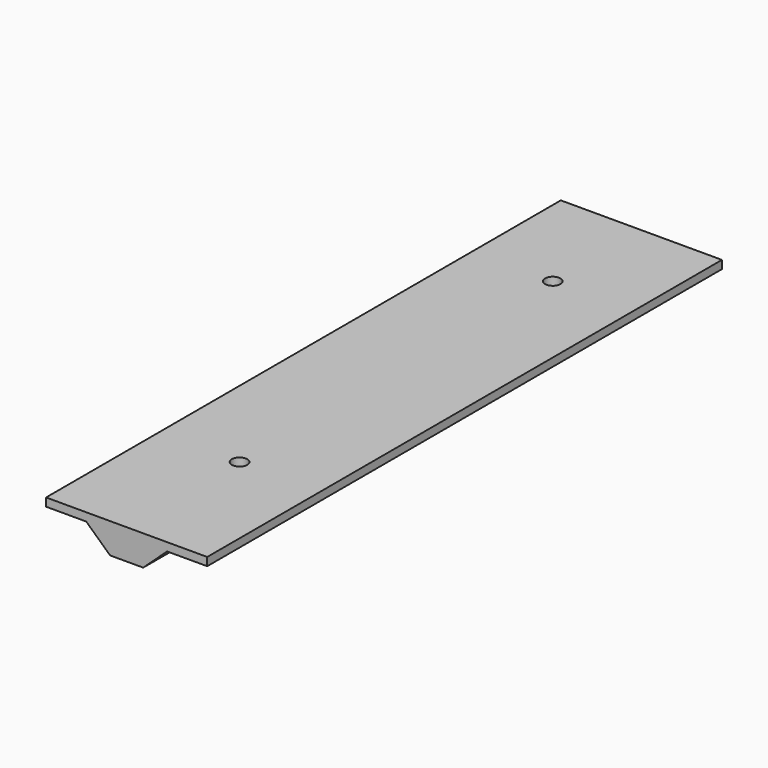
from build123d import *

# Parameters (mm, degrees)
F1_DEPTH = 175
F2_R     = 2.1
F3_DEPTH = 25
F4_DEPTH = 25
F5_DEPTH = 5
F6_DEPTH = 5


with BuildPart() as f1:
    # F0 (on Front) → F1 (new body)
    with BuildSketch(Plane.XZ):
        Polygon((4.5, 4), (11, 10), (-11, 10), (-4.5, 4), (0, 4), align=None)
        Polygon((11, 10), (21.9141976312, 10), (21.9141976312, 12.2224409133), (-21.9141976312, 12.2224409133), (-21.9141976312, 10), (-11, 10), align=None)
    extrude(amount=F1_DEPTH)

    # F2 (on face) → F3 (cut)
    with BuildSketch(Plane(origin=(0, 0, 4), x_dir=(1, 0, 0), z_dir=(0, 0, -1))):
        with Locations((0, 136.6154402494)):
            Circle(F2_R)
    extrude(amount=-F3_DEPTH, mode=Mode.SUBTRACT)

    # F2 (on face) → F4 (cut)
    with BuildSketch(Plane(origin=(0, 0, 4), x_dir=(1, 0, 0), z_dir=(0, 0, -1))):
        with Locations((0, 30.1199369133)):
            Circle(F2_R)
    extrude(amount=-F4_DEPTH, mode=Mode.SUBTRACT)

    # F2 (on face) → F5 (cut)
    with BuildSketch(Plane(origin=(0, 0, 4), x_dir=(1, 0, 0), z_dir=(0, 0, -1))):
        with BuildLine():
            ThreePointArc((4.5, 25.4295211534), (5.9791303716, 27.5704271565), (6.5, 30.1199369133))
            ThreePointArc((6.5, 30.1199369133), (5.9791303716, 32.66944667), (4.5, 34.8103526731))
            Line((4.5, 34.8103526731), (4.5, 25.4295211534))
        make_face()
        with BuildLine():
            Line((4.5, 25.4295211534), (4.5, 34.8103526731))
            ThreePointArc((4.5, 34.8103526731), (0, 36.6199369133), (-4.5, 34.8103526731))
            Line((-4.5, 34.8103526731), (-4.5, 25.4295211534))
            ThreePointArc((-4.5, 25.4295211534), (0, 23.6199369133), (4.5, 25.4295211534))
        make_face()
        with Locations((0, 30.1199369133)):
            Circle(F2_R, mode=Mode.SUBTRACT)
        with BuildLine():
            Line((-4.5, 25.4295211534), (-4.5, 34.8103526731))
            ThreePointArc((-4.5, 34.8103526731), (-6.5, 30.1199369133), (-4.5, 25.4295211534))
        make_face()
        with BuildLine():
            Line((4.5, 141.3058560093), (4.5, 131.9250244896))
            ThreePointArc((4.5, 131.9250244896), (5.9791303716, 134.0659304926), (6.5, 136.6154402494))
            ThreePointArc((6.5, 136.6154402494), (5.9791303716, 139.1649500062), (4.5, 141.3058560093))
        make_face()
    extrude(amount=-F5_DEPTH, mode=Mode.SUBTRACT)

    # F2 (on face) → F6 (cut)
    with BuildSketch(Plane(origin=(0, 0, 4), x_dir=(1, 0, 0), z_dir=(0, 0, -1))):
        with BuildLine():
            ThreePointArc((-4.5, 141.3058560093), (-6.5, 136.6154402494), (-4.5, 131.9250244896))
            Line((-4.5, 131.9250244896), (-4.5, 141.3058560093))
        make_face()
        with BuildLine():
            ThreePointArc((-4.5, 131.9250244896), (0, 130.1154402494), (4.5, 131.9250244896))
            Line((4.5, 131.9250244896), (4.5, 141.3058560093))
            ThreePointArc((4.5, 141.3058560093), (0, 143.1154402494), (-4.5, 141.3058560093))
            Line((-4.5, 141.3058560093), (-4.5, 131.9250244896))
        make_face()
        with Locations((0, 136.6154402494)):
            Circle(F2_R, mode=Mode.SUBTRACT)
    extrude(amount=-F6_DEPTH, mode=Mode.SUBTRACT)


solid = f1.part
